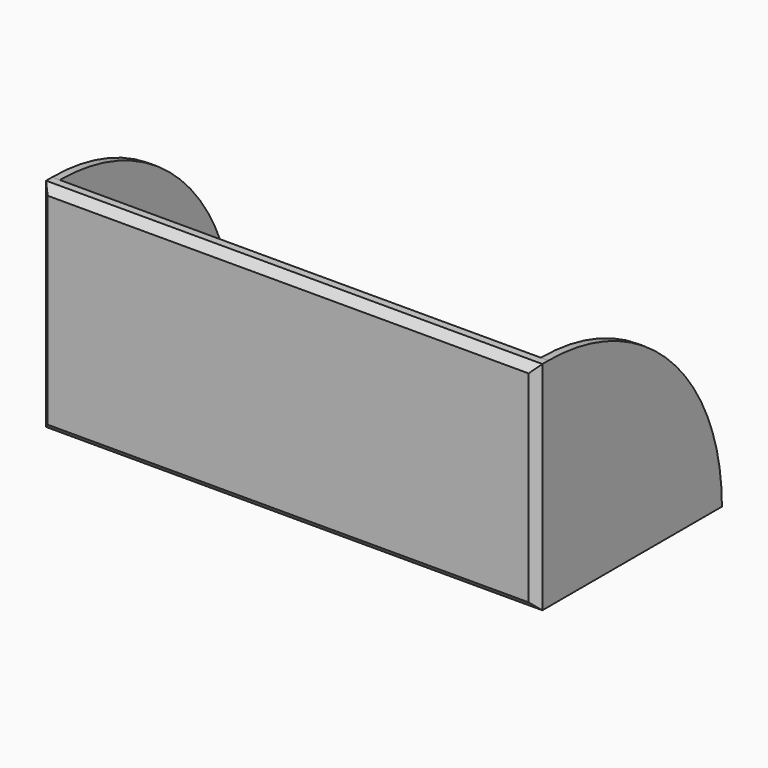
from build123d import *

# Parameters (mm, degrees)
F0_W     = 82.55
F0_H     = 36.068
F0_R     = 5.842
F1_DEPTH = 1.27
F2_W     = 1.27
F2_H     = 36.068
F3_DEPTH = 50.8
F5_DEPTH = 101.6
F6_W     = 80.01
F6_H     = 34.798
F7_DEPTH = 2.54
F9_SIZE  = 1.27


with BuildPart() as f1:
    # F0 (on Top) → F1 (new body)
    with BuildSketch(Plane.XY):
        with Locations((41.275, 18.034)):
            Rectangle(F0_W, F0_H)
        with Locations((8.89, 8.89)):
            Circle(F0_R, mode=Mode.SUBTRACT)
        with Locations((30.48, 8.89)):
            Circle(F0_R, mode=Mode.SUBTRACT)
        with Locations((52.07, 8.89)):
            Circle(F0_R, mode=Mode.SUBTRACT)
        with Locations((73.66, 8.89)):
            Circle(F0_R, mode=Mode.SUBTRACT)
        with Locations((8.89, 27.178)):
            Circle(F0_R, mode=Mode.SUBTRACT)
        with Locations((30.48, 27.178)):
            Circle(F0_R, mode=Mode.SUBTRACT)
        with Locations((52.07, 27.178)):
            Circle(F0_R, mode=Mode.SUBTRACT)
        with Locations((73.66, 27.178)):
            Circle(F0_R, mode=Mode.SUBTRACT)
    extrude(amount=F1_DEPTH)

    # F2 (on face) → F3 (join)
    with BuildSketch(Plane.XY.offset(1.27)):
        with Locations((0.635, 18.034)):
            Rectangle(F2_W, F2_H)
        with Locations((81.915, 18.034)):
            Rectangle(F2_W, F2_H)
    extrude(amount=F3_DEPTH)

    # F4 (on face) → F5 (cut)
    with BuildSketch(Plane(origin=(0, 0, 0), x_dir=(0, -1, 0), z_dir=(-1, 0, 0))):
        with BuildLine():
            Line((-36.068, 52.07), (-36.068, 0))
            ThreePointArc((-36.068, 0), (-25.5039273838, 25.5039273838), (0, 36.068))
            Line((0, 36.068), (0, 52.07))
            Line((0, 52.07), (-36.068, 52.07))
        make_face()
    extrude(amount=-F5_DEPTH, mode=Mode.SUBTRACT)


with BuildPart() as f7:
    # F6 (on face) → F7 (new body)
    with BuildSketch(Plane.XZ):
        with Locations((41.275, 18.669)):
            Rectangle(F6_W, F6_H)
        Polygon((0, 36.068), (0, 0), (82.55, 0), (82.55, 36.068), (81.28, 36.068), (81.28, 1.27), (1.27, 1.27), (1.27, 36.068), align=None)
    extrude(amount=F7_DEPTH)


with BuildPart() as f1_1:
    add(f1.part)

    # F8: union F7
    add(f7.part)

    # F9
    f9_edges = [f1_1.edges().sort_by_distance(p)[0] for p in [
        (82.55, -2.54, 18.034),
        (41.275, -2.54, 36.068),
        (41.275, -2.54, 0),
        (0, -2.54, 18.034),
    ]]
    chamfer(f9_edges, length=F9_SIZE)


solid = f1_1.part
